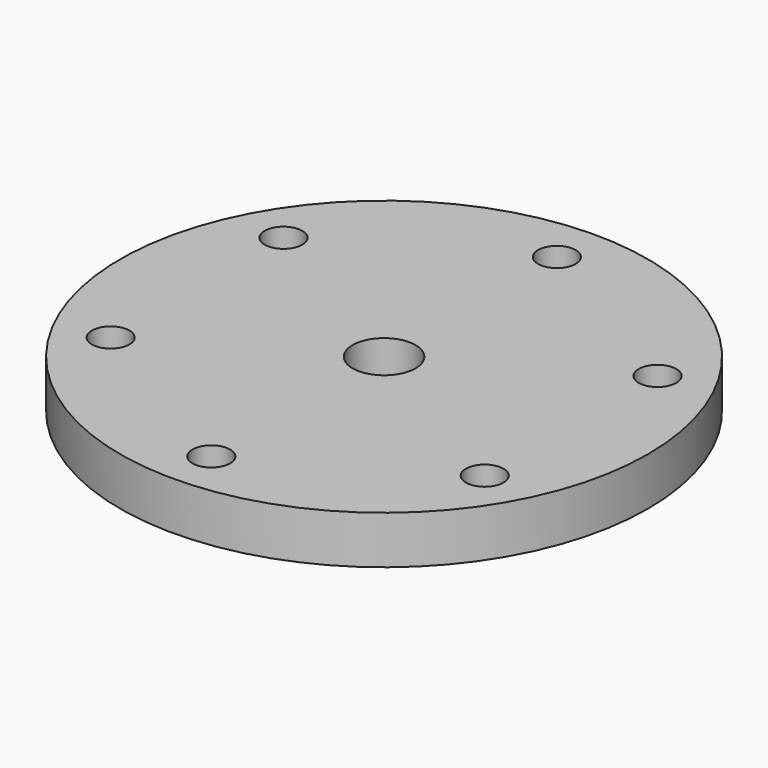
from build123d import *

# Parameters (mm, degrees)
F0_R            = 34.925
F1_DEPTH        = 6.35
F3_D            = 4.9784
F3_COPIES_COUNT = 6
F5_D            = 8.334375


# Not quite as in the source:
# - a pattern or mirror of a feature is missing from the dataset's text; its kind, count and spacing are read off the source's solid


with BuildPart() as f1:
    # F0 (on Top) → F1 (new body)
    with BuildSketch(Plane.XY):
        Circle(F0_R)
    extrude(amount=F1_DEPTH)

    # F3 (through all)
    with Locations(Plane.XY.offset(6.35)):
        with Locations((0, 28.575)):
            f3 = Hole(F3_D / 2)

    # F3_copies: F3 ×6 about axis
    f3_copies_axis = Axis((0, 0, 0), (0, 0, 1))
    for i in range(1, F3_COPIES_COUNT):
        add(f3.rotate(f3_copies_axis, i * 360 / F3_COPIES_COUNT), mode=Mode.SUBTRACT)

    # F5 (through all)
    with Locations(Plane.XY.offset(6.35)):
        with Locations((0, 0)):
            Hole(F5_D / 2)


solid = f1.part
